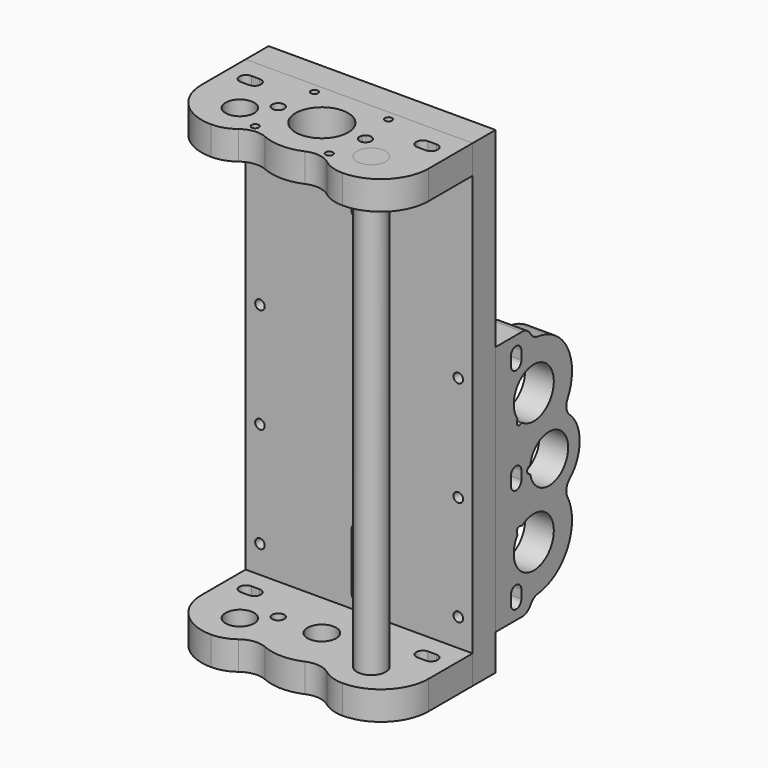
from build123d import *

# Parameters (mm, degrees)
F1_DEPTH       = 12
F2_R           = 11
F2_R_2         = 5.975
F3_DEPTH       = 12
F4_R           = 10
F5_R           = 6
F6_DEPTH       = 200
F8_DEPTH       = 12
F9_R           = 2.5
F9_R_2         = 6
F9_R_3         = 5.9749995874
F10_DEPTH      = 12
F11_R          = 2
F12_DEPTH      = 25
F12_DEPTH_BACK = 10
F13_R          = 1.5
F14_DEPTH      = 25
F15_R          = 5
F16_R          = 5


# Not quite as in the source:
# - ends of sketch curves that miss each other by under 0.0002 mm in the source are joined


with BuildPart() as f1:
    # F0 (on Front) → F1 (new body)
    with BuildSketch(Plane.XZ):
        Polygon((-47.5, 1.6334e-06), (47.5, -1.6334e-06), (47.5, 200.0000016334), (-47.5, 200.0000016334), align=None)
        with BuildLine():
            ThreePointArc((3.25, 18), (0, 14.75), (-3.25, 18))
            Line((-3.25, 18), (-3.25, 41))
            ThreePointArc((-3.25, 41), (0, 44.25), (3.25, 41))
            Line((3.25, 41), (3.25, 18))
        make_face(mode=Mode.SUBTRACT)
        with BuildLine():
            ThreePointArc((-3.25, 182.0000016334), (0, 185.2500016334), (3.25, 182.0000016334))
            Line((3.25, 182.0000016334), (3.25, 159.0000016334))
            ThreePointArc((3.25, 159.0000016334), (0, 155.7500016334), (-3.25, 159.0000016334))
            Line((-3.25, 159.0000016334), (-3.25, 182.0000016334))
        make_face(mode=Mode.SUBTRACT)
    extrude(amount=-F1_DEPTH)


with BuildPart() as f3:
    # F2 (on face) → F3 (new body)
    with BuildSketch(Plane.XY.offset(200.0000016334)):
        with BuildLine():
            Line((-7.7942286341, 0), (-47.5, 0))
            Line((-47.5, 0), (-47.5, -23))
            ThreePointArc((-47.5, -23), (-41.6421356237, -37.1421356237), (-27.5, -43))
            ThreePointArc((-27.5, -43), (-42.0543335736, -24.3707612055), (-20.4571797288, -14.7561832304))
            ThreePointArc((-20.4571797288, -14.7561832304), (-15.9364912858, -5.8241729502), (-7.7942286341, 0))
        make_face()
        with BuildLine():
            ThreePointArc((-38.75, -13.5), (-41.5, -10.75), (-38.75, -8))
            Line((-38.75, -8), (-35.25, -8))
            ThreePointArc((-35.25, -8), (-32.5, -10.75), (-35.25, -13.5))
            Line((-35.25, -13.5), (-38.75, -13.5))
        make_face(mode=Mode.SUBTRACT)
        with BuildLine():
            Line((7.7942286341, 0), (-7.7942286341, 0))
            ThreePointArc((-7.7942286341, 0), (-15.9364912858, -5.8241729502), (-20.4571797288, -14.7561832304))
            ThreePointArc((-20.4571797288, -14.7561832304), (-18.5664260205, -15.950466567), (-16.8742462967, -17.4125849124))
            ThreePointArc((-16.8742462967, -17.4125849124), (-16.4091811981, -17.8084367766), (-16.0539715251, -18.3052368697))
            ThreePointArc((-16.0539715251, -18.3052368697), (-13.4164914328, -22.8371726314), (-12.5, -28))
            ThreePointArc((-12.5, -28), (-12.9343908099, -31.5837171931), (-14.212403856, -34.9598698777))
            ThreePointArc((-14.212403856, -34.9598698777), (0, -40.5), (14.212403856, -34.9598698777))
            ThreePointArc((14.212403856, -34.9598698777), (12.5908669986, -26.3514390682), (16.0539715251, -18.3052368697))
            ThreePointArc((16.0539715251, -18.3052368697), (16.4091811981, -17.8084367766), (16.8742462967, -17.4125849124))
            ThreePointArc((16.8742462967, -17.4125849124), (18.5664260205, -15.950466567), (20.4571797288, -14.7561832304))
            ThreePointArc((20.4571797288, -14.7561832304), (15.9364912858, -5.8241729502), (7.7942286341, 0))
        make_face()
        with Locations((0, -19.5)):
            Circle(F2_R, mode=Mode.SUBTRACT)
        with BuildLine():
            Line((47.5, 0), (7.7942286341, 0))
            ThreePointArc((7.7942286341, 0), (15.9364912858, -5.8241729502), (20.4571797288, -14.7561832304))
            ThreePointArc((20.4571797288, -14.7561832304), (35.2252086034, -15.1422726723), (42.5, -28))
            ThreePointArc((42.5, -28), (38.1066017178, -38.6066017178), (27.5, -43))
            ThreePointArc((27.5, -43), (41.6421356237, -37.1421356237), (47.5, -23))
            Line((47.5, -23), (47.5, 0))
        make_face()
        with BuildLine():
            Line((38.75, -13.5), (35.25, -13.5))
            ThreePointArc((35.25, -13.5), (32.5, -10.75), (35.25, -8))
            Line((35.25, -8), (38.75, -8))
            ThreePointArc((38.75, -8), (41.5, -10.75), (38.75, -13.5))
        make_face(mode=Mode.SUBTRACT)
        with BuildLine():
            ThreePointArc((-16.8742462967, -17.4125849124), (-18.5664260205, -15.950466567), (-20.4571797288, -14.7561832304))
            ThreePointArc((-20.4571797288, -14.7561832304), (-20.0634554606, -25.7014316878), (-14.212403856, -34.9598698777))
            ThreePointArc((-14.212403856, -34.9598698777), (-12.9343908099, -31.5837171931), (-12.5, -28))
            ThreePointArc((-12.5, -28), (-13.4164914328, -22.8371726314), (-16.0539715251, -18.3052368697))
            ThreePointArc((-16.0539715251, -18.3052368697), (-15.8271843666, -18.8835874706), (-15.75, -19.5))
            ThreePointArc((-15.75, -19.5), (-20.4510661347, -20.6854568195), (-16.8742462967, -17.4125849124))
        make_face()
        with BuildLine():
            ThreePointArc((-14.212403856, -34.9598698777), (-20.0634554606, -25.7014316878), (-20.4571797288, -14.7561832304))
            ThreePointArc((-20.4571797288, -14.7561832304), (-42.0543335736, -24.3707612055), (-27.5, -43))
            ThreePointArc((-27.5, -43), (-19.7346296986, -40.8335117595), (-14.212403856, -34.9598698777))
        make_face()
        with Locations((-27.5, -28)):
            Circle(F2_R_2, mode=Mode.SUBTRACT)
        with BuildLine():
            ThreePointArc((42.5, -28), (35.2252086034, -15.1422726723), (20.4571797288, -14.7561832304))
            ThreePointArc((20.4571797288, -14.7561832304), (20.0634554606, -25.7014316878), (14.212403856, -34.9598698777))
            ThreePointArc((14.212403856, -34.9598698777), (19.7346296986, -40.8335117595), (27.5, -43))
            ThreePointArc((27.5, -43), (38.1066017178, -38.6066017178), (42.5, -28))
        make_face()
        with Locations((27.5, -28)):
            Circle(F2_R_2, mode=Mode.SUBTRACT)
        with BuildLine():
            ThreePointArc((14.212403856, -34.9598698777), (20.0634554606, -25.7014316878), (20.4571797288, -14.7561832304))
            ThreePointArc((20.4571797288, -14.7561832304), (18.5664260205, -15.950466567), (16.8742462967, -17.4125849124))
            ThreePointArc((16.8742462967, -17.4125849124), (19.4354568195, -17.2989338653), (20.75, -19.5))
            ThreePointArc((20.75, -19.5), (17.6335874706, -21.9228156334), (16.0539715251, -18.3052368697))
            ThreePointArc((16.0539715251, -18.3052368697), (12.5908669986, -26.3514390682), (14.212403856, -34.9598698777))
        make_face()
    extrude(amount=-F3_DEPTH)

    # F4
    f4_edges = [f3.edges().sort_by_distance(p)[0] for p in [
        (-14.212404, -34.95987, 194.000002),
        (14.212404, -34.95987, 194.000002),
    ]]
    fillet(f4_edges, radius=F4_R)


with BuildPart() as f6:
    # F5 (on face) → F6 (new body)
    with BuildSketch(Plane.XY.offset(200.0000016334)):
        with Locations((27.5, -28)):
            Circle(F5_R)
    extrude(amount=-F6_DEPTH)


with BuildPart() as f8:
    # F7 (on face) → F8 (new body)
    with BuildSketch(Plane.YZ.offset(47.5)):
        with BuildLine():
            Line((28.5, 14.9999964573), (32, 19.9999983666))
            ThreePointArc((32, 19.9999983666), (46.1421356237, 25.8578627429), (52, 39.9999983666))
            ThreePointArc((52, 39.9999983666), (50.7273420335, 47.0204442471), (47.071333964, 53.1474274897))
            ThreePointArc((47.071333964, 53.1474274897), (56, 67.4999964573), (47.071333964, 81.8525654249))
            ThreePointArc((47.071333964, 81.8525654249), (50.7273420335, 87.9795486675), (52, 94.9999945479))
            ThreePointArc((52, 94.9999945479), (46.1421356237, 109.1421301717), (32, 114.9999945479))
            Line((32, 114.9999945479), (28.5, 119.9999964573))
            Line((28.5, 119.9999964573), (12, 119.9999964573))
            Line((12, 119.9999964573), (12, 14.9999964573))
            Line((12, 14.9999964573), (28.5, 14.9999964573))
        make_face()
        with BuildLine():
            ThreePointArc((20, 25.2499964573), (22.75, 27.9999964573), (25.5, 25.2499964573))
            Line((25.5, 25.2499964573), (25.5, 21.7499964573))
            ThreePointArc((25.5, 21.7499964573), (22.75, 18.9999964573), (20, 21.7499964573))
            Line((20, 21.7499964573), (20, 25.2499964573))
        make_face(mode=Mode.SUBTRACT)
        with BuildLine():
            ThreePointArc((26.2943182564, 48.7846907824), (39.4069435329, 32.5930548337), (23.2153075842, 45.7056801102))
            ThreePointArc((23.2153075842, 45.7056801102), (23.3755438907, 46.2028582229), (23.2632266648, 46.7130019187))
            ThreePointArc((23.2632266648, 46.7130019187), (23.5323962953, 48.4676020713), (25.286996448, 48.7367717018))
            ThreePointArc((25.286996448, 48.7367717018), (25.7971401438, 48.6244544759), (26.2943182564, 48.7846907824))
        make_face(mode=Mode.SUBTRACT)
        with BuildLine():
            Line((20, 65.5727162957), (20, 69.0727162957))
            ThreePointArc((20, 69.0727162957), (22.75, 71.8227162957), (25.5, 69.0727162957))
            Line((25.5, 69.0727162957), (25.5, 65.5727162957))
            ThreePointArc((25.5, 65.5727162957), (22.75, 62.8227162957), (20, 65.5727162957))
        make_face(mode=Mode.SUBTRACT)
        with BuildLine():
            ThreePointArc((30.2641799544, 69.6712709771), (49.975, 67.4999964573), (30.2641799544, 65.3287219374))
            ThreePointArc((30.2641799544, 65.3287219374), (30.0228916348, 65.7894059146), (29.5828947368, 66.0666287667))
            ThreePointArc((29.5828947368, 66.0666287667), (28.525, 67.4999964573), (29.5828947368, 68.9333641478))
            ThreePointArc((29.5828947368, 68.9333641478), (30.0228916348, 69.210587), (30.2641799544, 69.6712709771))
        make_face(mode=Mode.SUBTRACT)
        with BuildLine():
            Line((25.5, 113.2499964573), (25.5, 109.7499964573))
            ThreePointArc((25.5, 109.7499964573), (22.75, 106.9999964573), (20, 109.7499964573))
            Line((20, 109.7499964573), (20, 113.2499964573))
            ThreePointArc((20, 113.2499964573), (22.75, 115.9999964573), (25.5, 113.2499964573))
        make_face(mode=Mode.SUBTRACT)
        with BuildLine():
            ThreePointArc((23.2632266648, 88.2869909959), (23.3755438907, 88.7971346917), (23.2153075842, 89.2943128043))
            ThreePointArc((23.2153075842, 89.2943128043), (39.4069435329, 102.4069380809), (26.2943182564, 86.2153021321))
            ThreePointArc((26.2943182564, 86.2153021321), (25.7971401438, 86.3755384387), (25.286996448, 86.2632212128))
            ThreePointArc((25.286996448, 86.2632212128), (23.5323962953, 86.5323908432), (23.2632266648, 88.2869909959))
        make_face(mode=Mode.SUBTRACT)
    extrude(amount=-F8_DEPTH)


with BuildPart() as f10:
    # F9 (on face) → F10 (new body)
    with BuildSketch(Plane(origin=(0, 0, 0), x_dir=(1, 0, -3.44e-08), z_dir=(-3.44e-08, 0, -1))):
        with BuildLine():
            Line((-47.5000064647, 23), (-47.5000064647, 0))
            Line((-47.5000064647, 0), (47.4999935353, 0))
            Line((47.4999935353, 0), (47.4999935353, 23))
            ThreePointArc((47.4999935353, 23), (41.642129159, 37.1421356237), (27.4999935353, 43))
            ThreePointArc((27.4999935353, 43), (22.7171729837, 42.217054249), (18.4336446722, 39.9499508691))
            ThreePointArc((18.4336446722, 39.9499508691), (13.5760954684, 37.9872452657), (8.3928255173, 38.7499445297))
            ThreePointArc((8.3928255173, 38.7499445297), (-6.8774e-06, 40.5), (-8.392839272, 38.7499445297))
            ThreePointArc((-8.392839272, 38.7499445297), (-13.5761092231, 37.9872452657), (-18.4336584269, 39.9499508691))
            ThreePointArc((-18.4336584269, 39.9499508691), (-22.7171867384, 42.217054249), (-27.5000068774, 43))
            ThreePointArc((-27.5000068774, 43), (-41.6421420885, 37.1421356237), (-47.5000064647, 23))
        make_face()
        with BuildLine():
            Line((-35.2500064647, 8), (-38.7500064647, 8))
            ThreePointArc((-38.7500064647, 8), (-41.5000064647, 10.75), (-38.7500064647, 13.5))
            Line((-38.7500064647, 13.5), (-35.2500064647, 13.5))
            ThreePointArc((-35.2500064647, 13.5), (-32.5000064647, 10.75), (-35.2500064647, 8))
        make_face(mode=Mode.SUBTRACT)
        with Locations((-18.2500068774, 19.5)):
            Circle(F9_R, mode=Mode.SUBTRACT)
        with Locations((-6.8774e-06, 19.5)):
            Circle(F9_R_2, mode=Mode.SUBTRACT)
        with Locations((18.2499931226, 19.5)):
            Circle(F9_R, mode=Mode.SUBTRACT)
        with BuildLine():
            ThreePointArc((35.2499935353, 8), (32.4999935353, 10.75), (35.2499935353, 13.5))
            Line((35.2499935353, 13.5), (38.7499935353, 13.5))
            ThreePointArc((38.7499935353, 13.5), (41.4999935353, 10.75), (38.7499935353, 8))
            Line((38.7499935353, 8), (35.2499935353, 8))
        make_face(mode=Mode.SUBTRACT)
        with Locations((-27.5000068774, 28)):
            Circle(F9_R_3, mode=Mode.SUBTRACT)
        with Locations((27.4999931226, 28)):
            Circle(F9_R_3, mode=Mode.SUBTRACT)
    extrude(amount=-F10_DEPTH)


with BuildPart() as f12_tool:
    # F11 (on face) → F12 (new body, two sides)
    with BuildSketch(Plane(origin=(0, 12, 0), x_dir=(-1, 0, 0), z_dir=(0, 1, 0))) as f12_sk:
        with Locations((-37, 194.0000016334)):
            Circle(F11_R)
        with Locations((37, 194.0000016334)):
            Circle(F11_R)
        with Locations((37, 6.0000016334)):
            Circle(F11_R)
        with Locations((-37, 6.0000016334)):
            Circle(F11_R)
        with Locations((-41.5, 23.4999987879)):
            Circle(F11_R)
        with Locations((-41.5, 111.4999987879)):
            Circle(F11_R)
        with Locations((-41.5, 67.4999987879)):
            Circle(F11_R)
        with Locations((41.5, 23.4999987879)):
            Circle(F11_R)
        with Locations((41.5, 111.4999987879)):
            Circle(F11_R)
        with Locations((41.5, 67.4999987879)):
            Circle(F11_R)
    extrude(amount=-F12_DEPTH)
    extrude(f12_sk.sketch, amount=F12_DEPTH_BACK)


with BuildPart() as f1_1:
    add(f1.part)

    # F12: cut by f12_tool
    add(f12_tool.part, mode=Mode.SUBTRACT)


with BuildPart() as f3_1:
    add(f3.part)

    # F12: cut by f12_tool
    add(f12_tool.part, mode=Mode.SUBTRACT)

    # F13 (on face) → F14 (cut)
    with BuildSketch(Plane.XY.offset(200.0000016334)):
        with Locations((-15.5, -4)):
            Circle(F13_R)
        with Locations((-15.5, -35)):
            Circle(F13_R)
        with Locations((15.5, -35)):
            Circle(F13_R)
        with Locations((15.5, -4)):
            Circle(F13_R)
    extrude(amount=-F14_DEPTH, mode=Mode.SUBTRACT)


with BuildPart() as f8_1:
    add(f8.part)

    # F12: cut by f12_tool
    add(f12_tool.part, mode=Mode.SUBTRACT)

    # F15
    f15_edges = [f8_1.edges().sort_by_distance(p)[0] for p in [
        (41.5, 32, 19.999998),
        (41.5, 28.5, 14.999996),
        (41.5, 32, 114.999995),
        (41.5, 28.5, 119.999996),
    ]]
    fillet(f15_edges, radius=F15_R)

    # F16
    f16_edges = [f8_1.edges().sort_by_distance(p)[0] for p in [
        (41.5, 47.071334, 81.852565),
        (41.5, 47.071334, 53.147427),
    ]]
    fillet(f16_edges, radius=F16_R)


with BuildPart() as f10_1:
    add(f10.part)

    # F12: cut by f12_tool
    add(f12_tool.part, mode=Mode.SUBTRACT)


solid = Compound([f6.part, f1_1.part, f3_1.part, f8_1.part, f10_1.part])
